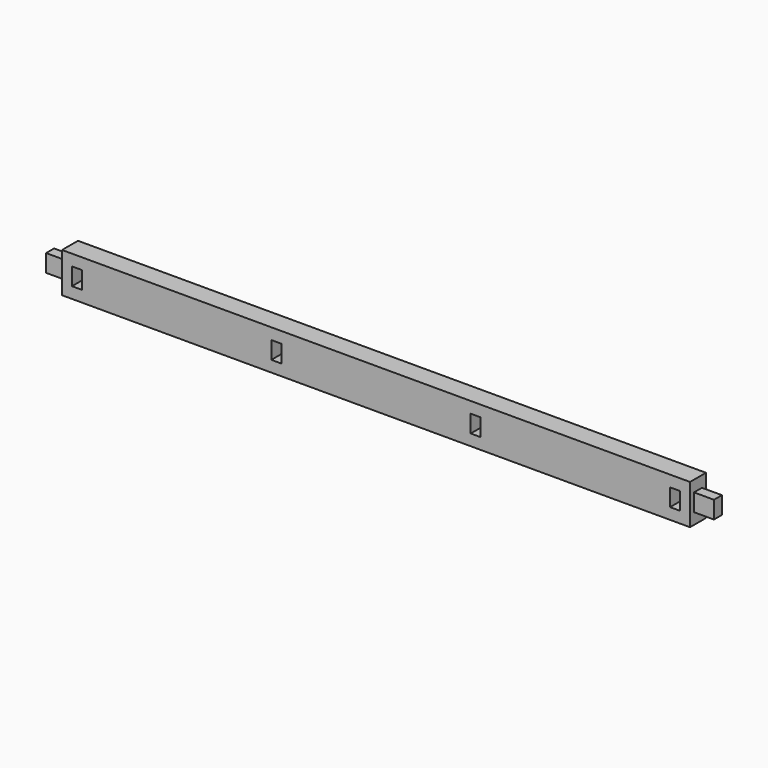
from build123d import *

# Parameters (mm, degrees)
F0_W     = 50.8
F0_H     = 101.6
F1_DEPTH = 850.9
F2_W     = 50.8
F2_H     = 101.6
F2_W_2   = 25.4
F2_H_2   = 44.45
F3_DEPTH = 50.8
F4_W     = 25.4
F4_H     = 44.45
F5_DEPTH = 50.801


# Not quite as in the source:
# - a pattern or mirror of a feature is missing from the dataset's text; its kind, count and spacing are read off the source's solid


with BuildPart() as f1:
    # F0 (on Right) → F1 (new body, symmetric)
    with BuildSketch(Plane.YZ):
        Rectangle(F0_W, F0_H)
    extrude(amount=F1_DEPTH, both=True)

    # F2 (on face) → F3 (cut)
    with BuildSketch(Plane(origin=(-850.9, 0, 0), x_dir=(0, -1, 0), z_dir=(-1, 0, 0))):
        Rectangle(F2_W, F2_H)
        Rectangle(F2_W_2, F2_H_2, mode=Mode.SUBTRACT)
    f3 = extrude(amount=-F3_DEPTH, mode=Mode.SUBTRACT)

    # F3_copies: F3 across plane
    add(f3.mirror(Plane(origin=(0, 0, 0), x_dir=(0, 0, 1), z_dir=(1, 0, 0))), mode=Mode.SUBTRACT)

    # F4 (on face) → F5 (cut, through all)
    with BuildSketch(Plane.XZ.offset(25.4)):
        with Locations((-762, 0)):
            Rectangle(F4_W, F4_H)
        with Locations((-254, 0)):
            Rectangle(F4_W, F4_H)
    f5 = extrude(amount=-F5_DEPTH, mode=Mode.SUBTRACT)

    # F5_copies: F5 across plane
    add(f5.mirror(Plane(origin=(0, 0, 0), x_dir=(0, 0, 1), z_dir=(1, 0, 0))), mode=Mode.SUBTRACT)


solid = f1.part
